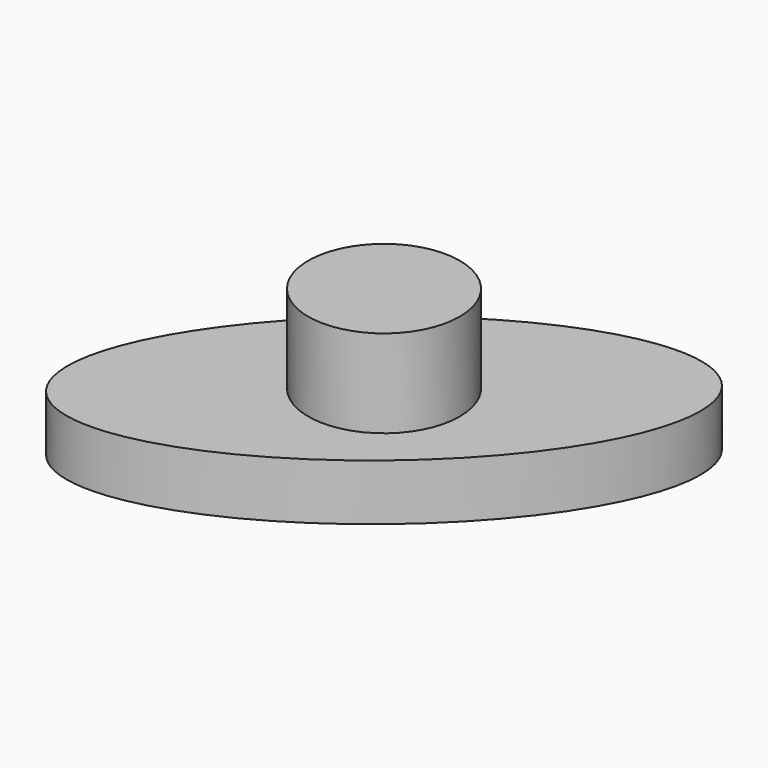
from build123d import *

# Parameters (mm, degrees)
F0_R      = 12.7
F1_DEPTH  = 14.732
F1_FACE_R = 12.7
F3_DEPTH  = 9.4


# Not quite as in the source:
# - the program builds the solid bodies; features that only make, move or delete a surface that nothing else refers to are left out


with BuildPart() as f1:
    # F0 (on Top) → F1 (new body)
    with BuildSketch(Plane.XY):
        with Locations((0.2708127431, 0.1451327698)):
            Circle(F0_R)
    extrude(amount=F1_DEPTH)

    # F0 (on Top) + F1_face (on face) → F3 (join)
    with BuildSketch(Plane.XY):
        with BuildLine():
            add(Edge.make_bspline(
                [(-33.6368591517, -28.2527666673), (-10.9653906557, -55.322963068), (28.5603829384, 0.8089842881), (68.0861565326, 56.9409316442), (5.8889144425, 27.8791806888), (-56.3083276476, -1.1825702666), (-33.6368591517, -28.2527666673)],
                knots=[0, 0, 0, 2.0943951024, 2.0943951024, 4.1887902048, 4.1887902048, 6.2831853072, 6.2831853072, 6.2831853072], degree=2, weights=[1, 0.5, 1, 0.5, 1, 0.5, 1]))
        make_face()
        with Locations((0.2708127431, 0.1451327698)):
            Circle(F0_R, mode=Mode.SUBTRACT)
    with BuildSketch(Plane(origin=(0.2708127431, 0.1451327698, 14.732), x_dir=(1, 0, 0), z_dir=(0, 0, 1))):
        Circle(F1_FACE_R)
    extrude(amount=-F3_DEPTH)


solid = f1.part
